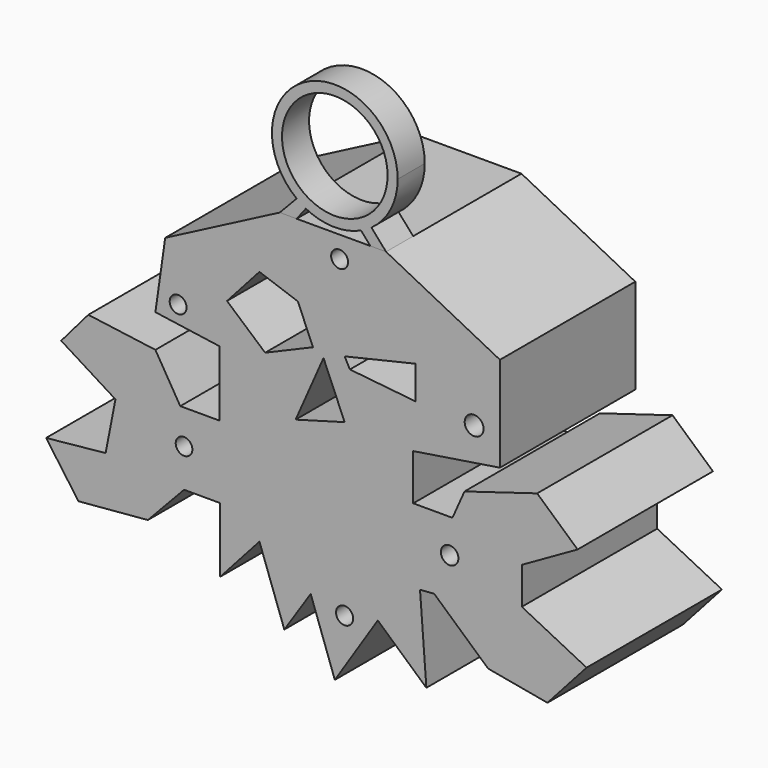
from build123d import *

# Parameters (mm, degrees)
F0_R     = 0.6253308063
F0_R_2   = 0.6576470557
F0_R_3   = 0.6430310393
F0_R_4   = 0.6325864549
F0_R_5   = 0.7087084558
F0_R_6   = 0.63416899
F1_DEPTH = 12.7
F3_R     = 3.9624414974
F4_DEPTH = 2.54


# Not quite as in the source:
# - the program builds the solid bodies; features that only make, move or delete a surface that nothing else refers to are left out


with BuildPart() as f1:
    # F0 (on Front) → F1 (new body)
    with BuildSketch(Plane.XZ):
        Polygon((-61.8477277458, 13.6200906709), (-63.8848692179, 11.2434281036), (-59.810589999, 8.6970031261), (-60.5462230742, 4.9056601711), (-65.0166124105, 4.4529624283), (-62.5833645463, 1.0577295907), (-57.3773384094, 1.5104275662), (-54.661154747, 4.3963752687), (-53.1898848712, 4.3963752687), (-53.1898848712, 9.8287472501), (-54.9440905452, 9.8287472501), (-56.8114668131, 12.941043824), align=None)
        with Locations((-54.6610355377, 7.2603821754)):
            Circle(F0_R, mode=Mode.SUBTRACT)
        Polygon((-34.516107291, 9.0931132436), (-35.9873734415, 9.0931132436), (-35.8845129038, 3.6278230993), (-31.8380962585, 0), (-27.3861158639, -0.8096481324), (-24.4493998371, 2.4659185885), (-29.3100811541, 4.9056601711), (-29.3100811541, 7.6784333214), (-25.1226276159, 10.0550958887), (-28.1569631866, 12.7755356355), (-33.6107090116, 11.1302537844), align=None)
        with Locations((-34.7257182002, 6.5483227372)):
            Circle(F0_R_2, mode=Mode.SUBTRACT)
        Polygon((-52.0185305594, 9.8287472501), (-53.1898848712, 9.8287472501), (-53.1898848712, 4.3963752687), (-51.9449673593, 4.3963752687), (-51.9449673593, -0.4701253201), (-49.0024313331, 2.8119329363), (-47.1350550652, -2.3940897081), (-45.1545007527, 0.6050316733), (-43.3437116444, -4.4878176413), (-40.11823982, 0.4918571794), (-36.4727111343, -2.7765490017), (-36.9493551552, 3.54756671), (-35.8845129038, 3.6278230993), (-35.9873734415, 9.0931132436), (-37.4586395919, 9.0931132436), (-37.4586395919, 12.5449337065), (-30.9511106461, 13.5635035113), (-30.9511106461, 20.6934921443), (-39.495781064, 25.0507071614), (-47.474578023, 25.0507071614), (-56.0758337379, 20.5803178251), (-56.8114668131, 15.4308816418), (-52.0185305594, 14.7461770819), align=None)
        with Locations((-42.6119677722, 0)):
            Circle(F0_R_3, mode=Mode.SUBTRACT)
        with Locations((-55.1074296236, 16.4904613048)):
            Circle(F0_R_4, mode=Mode.SUBTRACT)
        Polygon((-48.5752017703, 15.4308816418), (-51.4356829226, 17.9207194597), (-49.0024313331, 20.6347298909), (-46.1164824665, 19.6183361113), (-44.9847392738, 16.9587358832), align=None, mode=Mode.SUBTRACT)
        Polygon((-42.6080785692, 12.7825982869), (-46.2862439454, 11.7527125403), (-44.1925190389, 16.5060386062), align=None, mode=Mode.SUBTRACT)
        Polygon((-42.2119647264, 16.3928642869), (-42.6080785692, 17.1284973621), (-37.288878113, 18.3734167367), (-37.288878113, 15.8835798502), align=None, mode=Mode.SUBTRACT)
        with Locations((-32.8873321414, 15.7226305455)):
            Circle(F0_R_5, mode=Mode.SUBTRACT)
        with Locations((-42.985662818, 23.4314408153)):
            Circle(F0_R_6, mode=Mode.SUBTRACT)
    extrude(amount=F1_DEPTH)


with BuildPart() as f4:
    # F3 (on face) → F4 (new body)
    with BuildSketch(Plane.XZ.offset(12.7)):
        with BuildLine():
            ThreePointArc((-40.5978600179, 26.2984021236), (-39.1484875063, 27.9782117542), (-38.6269349154, 30.1346959223))
            ThreePointArc((-38.6269349154, 30.1346959223), (-45.437652272, 34.3648308471), (-46.2107199183, 26.3847131282))
            ThreePointArc((-46.2107199183, 26.3847131282), (-45.8743308801, 26.1501557938), (-45.5188478641, 25.9456892843))
            ThreePointArc((-45.5188478641, 25.9456892843), (-43.4592958766, 25.4170304905), (-41.3767340339, 25.8461816066))
            ThreePointArc((-41.3767340339, 25.8461816066), (-40.9764839308, 26.053668122), (-40.5978600179, 26.2984021236))
        make_face()
        with Locations((-43.3459614898, 30.1346959223)):
            Circle(F3_R, mode=Mode.SUBTRACT)
        with BuildLine():
            Line((-46.2107199183, 26.3847131282), (-47.474578023, 25.0507071614))
            Line((-47.474578023, 25.0507071614), (-46.2107199183, 25.0507071614))
            Line((-46.2107199183, 25.0507071614), (-45.5188478641, 25.9456892843))
            ThreePointArc((-45.5188478641, 25.9456892843), (-45.8743308801, 26.1501557938), (-46.2107199183, 26.3847131282))
        make_face()
        with BuildLine():
            Line((-41.3767340339, 25.8461816066), (-40.674097836, 25.0507071614))
            Line((-40.674097836, 25.0507071614), (-39.495781064, 25.0507071614))
            Line((-39.495781064, 25.0507071614), (-40.5978600179, 26.2984021236))
            ThreePointArc((-40.5978600179, 26.2984021236), (-40.9764839308, 26.053668122), (-41.3767340339, 25.8461816066))
        make_face()
    extrude(amount=-F4_DEPTH)


solid = Compound([f1.part, f4.part])
